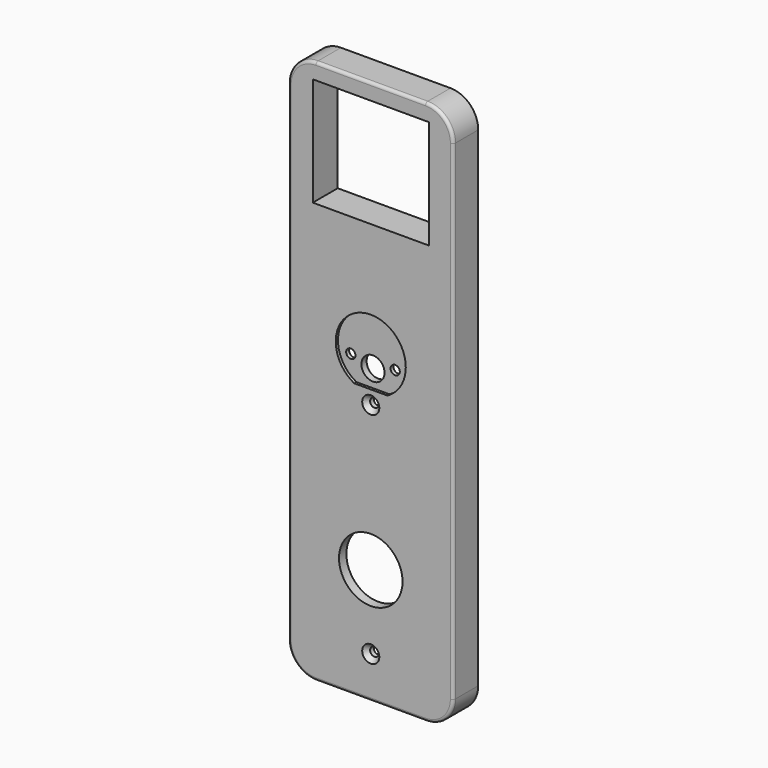
from build123d import *

# Parameters (mm, degrees)
F0_W           = 90.678
F0_H           = 217.4875
F1_DEPTH       = 17.145
F3_D           = 4.826
F3_CSINK_D     = 9.398
F3_CSINK_ANGLE = 84
F2_R           = 17.4625
F2_R_2         = 6.35
F2_R_3         = 2.54
F4_DEPTH       = 25.4
F5_W           = 77.978
F5_H           = 204.7875
F5_R           = 2.413
F5_R_2         = 17.4625
F5_R_3         = 6.35
F5_R_4         = 2.54
F6_DEPTH       = 12.065
F7_D           = 4.826
F7_CSINK_D     = 9.398
F7_CSINK_ANGLE = 84
F8_W           = 90.678
F8_H           = 81.915
F9_DEPTH       = 17.145
F10_W          = 63.754
F10_H          = 59.69
F11_DEPTH      = 17.146
F12_DEPTH      = 1.524
F13_W          = 9.525
F13_H          = 9.525
F13_R          = 2.54
F14_DEPTH      = 1.524
F15_R          = 5.08
F16_R          = 15.24
F17_R          = 1.5875


with BuildPart() as f1:
    # F0 (on Front) → F1 (new body)
    with BuildSketch(Plane.XZ):
        with Locations((45.339, 108.74375)):
            Rectangle(F0_W, F0_H)
    extrude(amount=F1_DEPTH)

    # F3 (through all)
    with Locations(Plane.XZ.offset(17.145)):
        with Locations((45.339, 22.86)):
            CounterSinkHole(F3_D / 2, F3_CSINK_D / 2, counter_sink_angle=F3_CSINK_ANGLE)

    # F2 (on face) → F4 (cut)
    with BuildSketch(Plane.XZ.offset(17.145)):
        with Locations((45.339, 63.5)):
            Circle(F2_R)
        with Locations((45.339, 160.3375)):
            Circle(F2_R_2)
        with Locations((33.147, 163.5125)):
            Circle(F2_R_3)
        with Locations((57.531, 163.5125)):
            Circle(F2_R_3)
    extrude(amount=-F4_DEPTH, mode=Mode.SUBTRACT)

    # F5 (on face) → F6 (cut)
    with BuildSketch(Plane(origin=(0, 0, 0), x_dir=(-1, 0, 0), z_dir=(0, 1, 0))):
        with Locations((-45.339, 108.74375)):
            Rectangle(F5_W, F5_H)
        with Locations((-45.339, 22.86)):
            Circle(F5_R, mode=Mode.SUBTRACT)
        with Locations((-45.339, 63.5)):
            Circle(F5_R_2, mode=Mode.SUBTRACT)
        with Locations((-45.339, 160.3375)):
            Circle(F5_R_3, mode=Mode.SUBTRACT)
        with Locations((-57.531, 163.5125)):
            Circle(F5_R_4, mode=Mode.SUBTRACT)
        with Locations((-33.147, 163.5125)):
            Circle(F5_R_4, mode=Mode.SUBTRACT)
    extrude(amount=-F6_DEPTH, mode=Mode.SUBTRACT)

    # F7 (through all)
    with Locations(Plane.XZ.offset(17.145)):
        with Locations((45.339, 143.3195)):
            CounterSinkHole(F7_D / 2, F7_CSINK_D / 2, counter_sink_angle=F7_CSINK_ANGLE)

    # F8 (on Front) → F9 (join, through all)
    with BuildSketch(Plane.XZ):
        with Locations((45.339, 258.445)):
            Rectangle(F8_W, F8_H)
    extrude(amount=F9_DEPTH)

    # F10 (on face) → F11 (cut, through all)
    with BuildSketch(Plane(origin=(0, 0, 0), x_dir=(-1, 0, 0), z_dir=(0, 1, 0))):
        with Locations((-45.339, 260.6675)):
            Rectangle(F10_W, F10_H)
    extrude(amount=-F11_DEPTH, mode=Mode.SUBTRACT)

    # F2 (on face) → F12 (cut)
    with BuildSketch(Plane.XZ.offset(17.145)):
        with BuildLine():
            ThreePointArc((54.4352503264, 150.8125), (61.8498032005, 157.8882238651), (64.5795, 167.767))
            ThreePointArc((64.5795, 167.767), (35.4602238651, 184.2778032005), (36.2427496736, 150.8125))
            Line((36.2427496736, 150.8125), (54.4352503264, 150.8125))
        make_face()
        with Locations((45.339, 160.3375)):
            Circle(F2_R_2, mode=Mode.SUBTRACT)
        with Locations((33.147, 163.5125)):
            Circle(F2_R_3, mode=Mode.SUBTRACT)
        with Locations((57.531, 163.5125)):
            Circle(F2_R_3, mode=Mode.SUBTRACT)
    extrude(amount=-F12_DEPTH, mode=Mode.SUBTRACT)

    # F13 (on face) → F14 (cut)
    with BuildSketch(Plane(origin=(0, -12.065, 0), x_dir=(-1, 0, 0), z_dir=(0, 1, 0))):
        with Locations((-57.531, 163.5125)):
            Rectangle(F13_W, F13_H)
        with Locations((-57.531, 163.5125)):
            Circle(F13_R, mode=Mode.SUBTRACT)
        with Locations((-33.147, 163.5125)):
            Rectangle(F13_W, F13_H)
        with Locations((-33.147, 163.5125)):
            Circle(F13_R, mode=Mode.SUBTRACT)
    extrude(amount=-F14_DEPTH, mode=Mode.SUBTRACT)

    # F15
    f15_edges = [f1.edges().sort_by_distance(p)[0] for p in [
        (84.328, -6.0325, 211.1375),
        (6.35, -6.0325, 211.1375),
        (6.35, -6.0325, 6.35),
        (84.328, -6.0325, 6.35),
    ]]
    fillet(f15_edges, radius=F15_R)

    # F16
    f16_edges = [f1.edges().sort_by_distance(p)[0] for p in [
        (90.678, -8.5725, 0),
        (0, -8.5725, 0),
        (0, -8.5725, 299.4025),
        (90.678, -8.5725, 299.4025),
    ]]
    fillet(f16_edges, radius=F16_R)

    # F17
    f17_edges = [f1.edges().sort_by_distance(p)[0] for p in [
        (0, -17.145, 149.70125),
        (45.339, -17.145, 0),
        (4.463693, -17.145, 4.463693),
        (86.214307, -17.145, 4.463693),
        (90.678, -17.145, 149.70125),
        (4.463693, -17.145, 294.938807),
        (86.214307, -17.145, 294.938807),
        (45.339, -17.145, 299.4025),
    ]]
    fillet(f17_edges, radius=F17_R)


solid = f1.part
